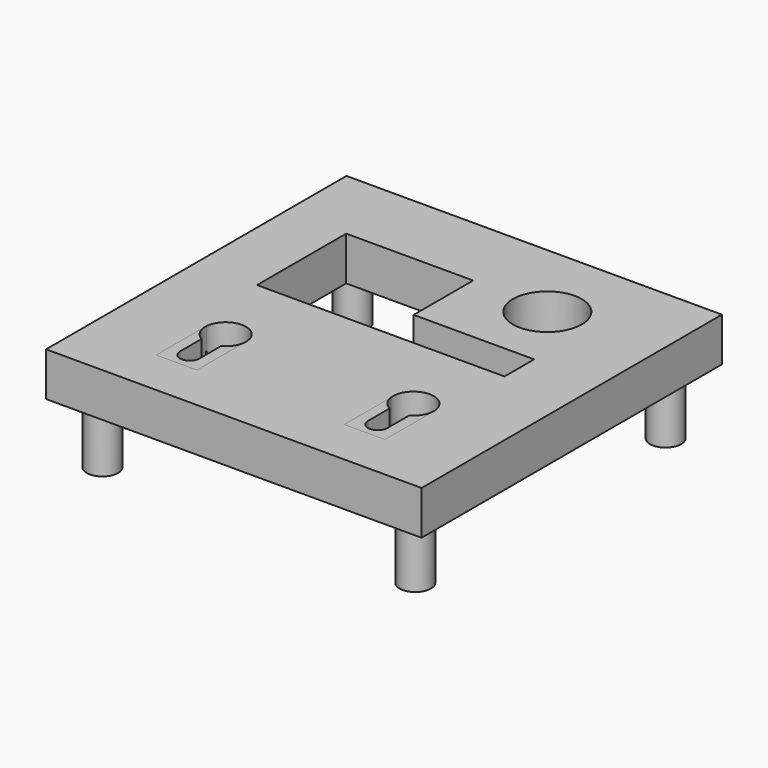
from build123d import *
from build123d import SkipClean  # not in build123d's __all__

# Parameters (mm, degrees)
F0_R     = 2.5
F1_DEPTH = 10
F0_W     = 60
F0_H     = 60
F0_R_2   = 5.5
F2_DEPTH = 7
F4_DEPTH = 25
F5_DEPTH = 10
F6_DEPTH = 3.5


with BuildPart() as f1:
    # F0 (on Top) → F1 (new body)
    with BuildSketch(Plane.XY):
        with Locations((-25, 25)):
            Circle(F0_R)
    extrude(amount=-F1_DEPTH)


with BuildPart() as f1b:
    # F0 (on Top) → F1, piece 2 (new body)
    with BuildSketch(Plane.XY):
        with Locations((25, 25)):
            Circle(F0_R)
    extrude(amount=-F1_DEPTH)


with BuildPart() as f1c:
    # F0 (on Top) → F1, piece 3 (new body)
    with BuildSketch(Plane.XY):
        with Locations((25, -25)):
            Circle(F0_R)
    extrude(amount=-F1_DEPTH)


with BuildPart() as f1d:
    # F0 (on Top) → F1, piece 4 (new body)
    with BuildSketch(Plane.XY):
        with Locations((-25, -25)):
            Circle(F0_R)
    extrude(amount=-F1_DEPTH)


with BuildPart() as f2:
    # F0 (on Top) → F2 (new body)
    with BuildSketch(Plane.XY):
        Rectangle(F0_W, F0_H)
        with Locations((-25, -25)):
            Circle(F0_R, mode=Mode.SUBTRACT)
        with Locations((25, -25)):
            Circle(F0_R, mode=Mode.SUBTRACT)
        Polygon((-20.2908944339, 5.9252767824), (-20.2908944339, 17.8066082299), (0, 17.8066082299), (0, 5.9252767824), (19.2535817623, 5.9252767824), (19.2535817623, 0), (0, 0), (-20.2908944339, 0), align=None, mode=Mode.SUBTRACT)
        with Locations((-25, 25)):
            Circle(F0_R, mode=Mode.SUBTRACT)
        with Locations((12.5, 17)):
            Circle(F0_R_2, mode=Mode.SUBTRACT)
        with Locations((25, 25)):
            Circle(F0_R, mode=Mode.SUBTRACT)
        with Locations((-25, 25)):
            Circle(F0_R)
        with Locations((-25, -25)):
            Circle(F0_R)
        with Locations((25, -25)):
            Circle(F0_R)
        with Locations((25, 25)):
            Circle(F0_R)
    extrude(amount=F2_DEPTH)

    # F3 (on face) → F4 (cut)
    with BuildSketch(Plane.XY.offset(7)):
        with BuildLine():
            Line((13.45, -20), (16.55, -20))
            ThreePointArc((16.55, -20), (15, -18.45), (13.45, -20))
        make_face()
        with BuildLine():
            ThreePointArc((13.45, -20), (15, -21.55), (16.55, -20))
            Line((16.55, -20), (13.45, -20))
        make_face()
        with BuildLine():
            ThreePointArc((13.45, -20), (15, -18.45), (16.55, -20))
            Line((16.55, -20), (16.55, -15.6721474181))
            Line((16.55, -15.6721474181), (16.5244984301, -15.6721474181))
            ThreePointArc((16.5244984301, -15.6721474181), (14.9905058647, -16.0716604569), (13.45, -15.6980489747))
            Line((13.45, -15.6980489747), (13.45, -20))
        make_face()
        with BuildLine():
            ThreePointArc((11.7551134899, -13.3424973788), (12.3250504464, -14.7199468679), (13.45, -15.6980489747))
            Line((13.45, -15.6980489747), (13.45, -15.6721474181))
            Line((13.45, -15.6721474181), (16.5244984301, -15.6721474181))
            ThreePointArc((16.5244984301, -15.6721474181), (17.7592810637, -14.4782844642), (18.2131267413, -12.8217757846))
            ThreePointArc((18.2131267413, -12.8217757846), (18.2116855273, -12.7249986477), (18.2073631634, -12.6283073425))
            Line((18.2073631634, -12.6283073425), (11.7551134899, -12.6283073425))
            Line((11.7551134899, -12.6283073425), (11.7551134899, -13.3424973788))
        make_face()
        with BuildLine():
            Line((13.45, -15.6721474181), (13.45, -15.6980489747))
            ThreePointArc((13.45, -15.6980489747), (14.9905058647, -16.0716604569), (16.5244984301, -15.6721474181))
            Line((16.5244984301, -15.6721474181), (13.45, -15.6721474181))
        make_face()
        with BuildLine():
            ThreePointArc((18.2073631634, -12.6283073425), (14.6055727154, -9.5915041058), (11.7551134899, -13.3424973788))
            Line((11.7551134899, -13.3424973788), (11.7551134899, -12.6283073425))
            Line((11.7551134899, -12.6283073425), (18.2073631634, -12.6283073425))
        make_face()
        with BuildLine():
            Line((-16.5981262033, -20), (-13.4981262033, -20))
            ThreePointArc((-13.4981262033, -20), (-15.0481262033, -18.45), (-16.5981262033, -20))
        make_face()
        with BuildLine():
            ThreePointArc((-16.5981262033, -20), (-15.0481262033, -21.55), (-13.4981262033, -20))
            Line((-13.4981262033, -20), (-16.5981262033, -20))
        make_face()
        with BuildLine():
            ThreePointArc((-16.5981262033, -20), (-15.0481262033, -18.45), (-13.4981262033, -20))
            Line((-13.4981262033, -20), (-13.4981262033, -15.678347156))
            ThreePointArc((-13.4981262033, -15.678347156), (-15.0481262033, -16.0717757846), (-16.5981262033, -15.678347156))
            Line((-16.5981262033, -15.678347156), (-16.5981262033, -20))
        make_face()
        with BuildLine():
            Line((-16.5981262033, -15.678347156), (-13.4981262033, -15.678347156))
            ThreePointArc((-13.4981262033, -15.678347156), (-12.3060093165, -14.5662800062), (-11.8038897812, -13.0152442266))
            Line((-11.8038897812, -13.0152442266), (-11.8038897812, -12.6283073425))
            Line((-11.8038897812, -12.6283073425), (-18.2923626253, -12.6283073425))
            ThreePointArc((-18.2923626253, -12.6283073425), (-17.8892283544, -14.3999514929), (-16.5981262033, -15.678347156))
        make_face()
        with BuildLine():
            ThreePointArc((-16.5981262033, -15.678347156), (-15.0481262033, -16.0717757846), (-13.4981262033, -15.678347156))
            Line((-13.4981262033, -15.678347156), (-16.5981262033, -15.678347156))
        make_face()
    extrude(amount=-F4_DEPTH, mode=Mode.SUBTRACT)

    # F3 (on face) → F5 (cut)
    with BuildSketch(Plane.XY.offset(7)):
        with BuildLine():
            Line((16.55, -15.6721474181), (16.55, -20))
            ThreePointArc((16.55, -20), (15, -21.55), (13.45, -20))
            Line((13.45, -20), (13.45, -15.6980489747))
            ThreePointArc((13.45, -15.6980489747), (12.3250504464, -14.7199468679), (11.7551134899, -13.3424973788))
            Line((11.7551134899, -13.3424973788), (11.7551134899, -22.6283073425))
            Line((11.7551134899, -22.6283073425), (18.2551134899, -22.6283073425))
            Line((18.2551134899, -22.6283073425), (18.2551134899, -12.6283073425))
            Line((18.2551134899, -12.6283073425), (18.2073631634, -12.6283073425))
            ThreePointArc((18.2073631634, -12.6283073425), (18.2116855273, -12.7249986477), (18.2131267413, -12.8217757846))
            ThreePointArc((18.2131267413, -12.8217757846), (17.7592810637, -14.4782844642), (16.5244984301, -15.6721474181))
            Line((16.5244984301, -15.6721474181), (16.55, -15.6721474181))
        make_face()
        with BuildLine():
            Line((-13.4981262033, -15.678347156), (-13.4981262033, -20))
            ThreePointArc((-13.4981262033, -20), (-15.0481262033, -21.55), (-16.5981262033, -20))
            Line((-16.5981262033, -20), (-16.5981262033, -15.678347156))
            ThreePointArc((-16.5981262033, -15.678347156), (-17.8892283544, -14.3999514929), (-18.2923626253, -12.6283073425))
            Line((-18.2923626253, -12.6283073425), (-18.3038897812, -12.6283073425))
            Line((-18.3038897812, -12.6283073425), (-18.3038897812, -22.6283073425))
            Line((-18.3038897812, -22.6283073425), (-11.8038897812, -22.6283073425))
            Line((-11.8038897812, -22.6283073425), (-11.8038897812, -13.0152442266))
            ThreePointArc((-11.8038897812, -13.0152442266), (-12.3060093165, -14.5662800062), (-13.4981262033, -15.678347156))
        make_face()
        with BuildLine():
            ThreePointArc((-11.8038897812, -12.6283073425), (-15.0481262033, -9.5717757846), (-18.2923626253, -12.6283073425))
            Line((-18.2923626253, -12.6283073425), (-11.8038897812, -12.6283073425))
        make_face()
    extrude(amount=-F5_DEPTH, mode=Mode.SUBTRACT)

    # F3 (on face) → F6 (join)
    with BuildSketch(Plane.XY.offset(7)):
        with BuildLine():
            Line((-13.4981262033, -15.678347156), (-13.4981262033, -20))
            ThreePointArc((-13.4981262033, -20), (-15.0481262033, -21.55), (-16.5981262033, -20))
            Line((-16.5981262033, -20), (-16.5981262033, -15.678347156))
            ThreePointArc((-16.5981262033, -15.678347156), (-17.8892283544, -14.3999514929), (-18.2923626253, -12.6283073425))
            Line((-18.2923626253, -12.6283073425), (-18.3038897812, -12.6283073425))
            Line((-18.3038897812, -12.6283073425), (-18.3038897812, -22.6283073425))
            Line((-18.3038897812, -22.6283073425), (-11.8038897812, -22.6283073425))
            Line((-11.8038897812, -22.6283073425), (-11.8038897812, -13.0152442266))
            ThreePointArc((-11.8038897812, -13.0152442266), (-12.3060093165, -14.5662800062), (-13.4981262033, -15.678347156))
        make_face()
        with BuildLine():
            Line((16.55, -15.6721474181), (16.55, -20))
            ThreePointArc((16.55, -20), (15, -21.55), (13.45, -20))
            Line((13.45, -20), (13.45, -15.6980489747))
            ThreePointArc((13.45, -15.6980489747), (12.3250504464, -14.7199468679), (11.7551134899, -13.3424973788))
            Line((11.7551134899, -13.3424973788), (11.7551134899, -22.6283073425))
            Line((11.7551134899, -22.6283073425), (18.2551134899, -22.6283073425))
            Line((18.2551134899, -22.6283073425), (18.2551134899, -12.6283073425))
            Line((18.2551134899, -12.6283073425), (18.2073631634, -12.6283073425))
            ThreePointArc((18.2073631634, -12.6283073425), (18.2116855273, -12.7249986477), (18.2131267413, -12.8217757846))
            ThreePointArc((18.2131267413, -12.8217757846), (17.7592810637, -14.4782844642), (16.5244984301, -15.6721474181))
            Line((16.5244984301, -15.6721474181), (16.55, -15.6721474181))
        make_face()
    with SkipClean():  # cleaning this boolean's faces spoils the solid; the shape is the same uncleaned
        extrude(amount=-F6_DEPTH)


solid = Compound([f1.part, f1b.part, f1c.part, f1d.part, f2.part])
